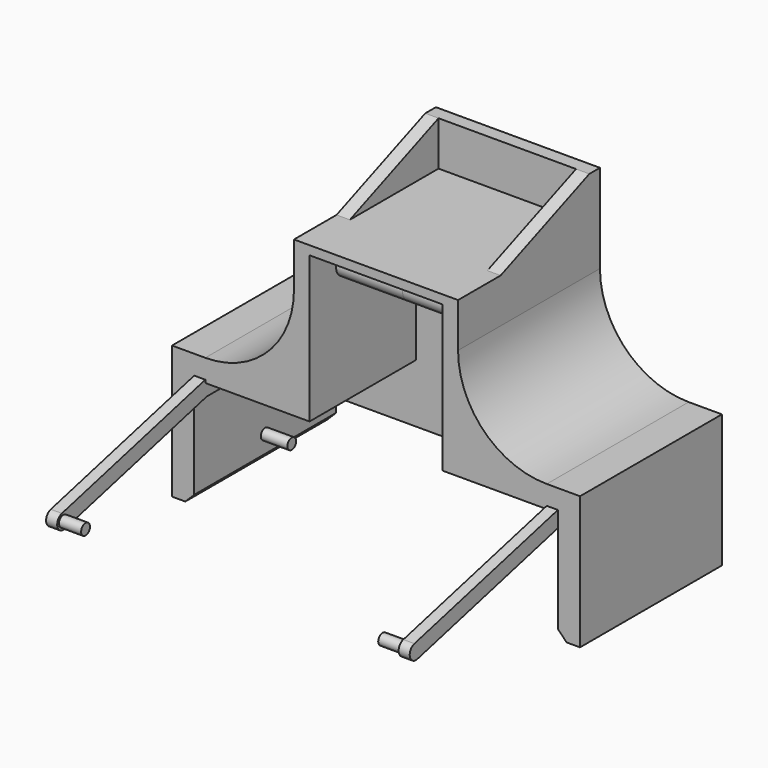
from build123d import *

# Parameters (mm, degrees)
F0_W          = 116.84
F0_H          = 76.2
F1_DEPTH      = 101.6
F3_DEPTH      = 76.2
F5_DEPTH      = 38.1
F5_DEPTH_BACK = 38.1
F6_R          = 3.1115
F7_DEPTH      = 114.3
F7_DEPTH_BACK = 114.3
F9_DEPTH      = 101.601
F11_DEPTH     = 25.401
F12_SIZE      = 5.08
F13_W         = 177.8
F13_H         = 62.1990481529
F14_DEPTH     = 76.2
F15_W         = 93.98
F15_H         = 7.62
F16_DEPTH     = 25.4
F18_DEPTH     = 7.62
F20_DEPTH     = 7.62
F21_R         = 3.175
F22_DEPTH     = 6.35
F23_DEPTH     = 19.05


with BuildPart() as f1:
    # F0 (on Front) → F1 (new body)
    with BuildSketch(Plane.XZ):
        with Locations((58.42, 38.1)):
            Rectangle(F0_W, F0_H)
        with Locations((-58.42, 38.1)):
            Rectangle(F0_W, F0_H)
        with Locations((58.42, -38.1)):
            Rectangle(F0_W, F0_H)
        with Locations((-58.42, -38.1)):
            Rectangle(F0_W, F0_H)
    extrude(amount=-F1_DEPTH)

    # F2 (on face) → F3 (cut)
    with BuildSketch(Plane.XZ):
        Polygon((-38.1, -12.7), (-104.14, -12.7), (-104.14, -69.85), (-104.14, -76.2), (104.14, -76.2), (104.14, -69.85), (104.14, -12.7), (38.1, -12.7), (38.1, 63.5), (-38.1, 63.5), align=None)
    extrude(amount=-F3_DEPTH, mode=Mode.SUBTRACT)

    # F4 (on Right) → F5 (cut, two sides)
    with BuildSketch(Plane.YZ) as f5_sk:
        Polygon((0, 71.12), (0, 63.5), (76.2, 63.5), align=None)
    extrude(amount=-F5_DEPTH, mode=Mode.SUBTRACT)
    extrude(f5_sk.sketch, amount=F5_DEPTH_BACK, mode=Mode.SUBTRACT)

    # F6 (on Right) → F7 (join, two sides)
    with BuildSketch(Plane.YZ) as f7_sk:
        with BuildLine():
            ThreePointArc((25.4005372305, 50.8), (29.8906652911, 52.6598719395), (31.7505372305, 57.15))
            ThreePointArc((31.7505372305, 57.15), (20.91040917, 61.6401280605), (25.4005372305, 50.8))
        make_face()
        with Locations((50.8005372305, -41.021)):
            Circle(F6_R)
        with Locations((50.8005372305, -61.087)):
            Circle(F6_R)
    extrude(amount=F7_DEPTH)
    extrude(f7_sk.sketch, amount=-F7_DEPTH_BACK)

    # F8 (on face) → F9 (cut, through all)
    with BuildSketch(Plane.XZ):
        with BuildLine():
            Line((-46.99, 76.2), (-116.84, 76.2))
            Line((-116.84, 76.2), (-116.84, 0))
            Line((-116.84, 0), (-97.79, 0))
            ThreePointArc((-97.79, 0), (-61.8689755157, 14.8789755157), (-46.99, 50.8))
            Line((-46.99, 50.8), (-46.99, 76.2))
        make_face()
        with BuildLine():
            Line((116.84, 0), (116.84, 76.2))
            Line((116.84, 76.2), (46.99, 76.2))
            Line((46.99, 76.2), (46.99, 50.8))
            ThreePointArc((46.99, 50.8), (61.8689755157, 14.8789755157), (97.79, 0))
            Line((97.79, 0), (116.84, 0))
        make_face()
    extrude(amount=-F9_DEPTH, mode=Mode.SUBTRACT)

    # F10 (on face) → F11 (cut, through all)
    with BuildSketch(Plane.XZ.offset(-76.2)):
        Polygon((104.14, -76.2), (104.14, -48.7679988146), (104.14, -46.2279988146), (-104.14, -46.2279988146), (-104.14, -48.7679988146), (-104.14, -76.2), align=None)
    extrude(amount=-F11_DEPTH, mode=Mode.SUBTRACT)

    # F12
    f12_edges = [f1.edges().sort_by_distance(p)[0] for p in [
        (104.14, 50.8, -76.2),
        (-104.14, 50.8, -76.2),
    ]]
    chamfer(f12_edges, length=F12_SIZE)

    # F13 (on Front) → F14 (cut)
    with BuildSketch(Plane.XZ):
        with Locations((0, -55.8045858206)):
            Rectangle(F13_W, F13_H)
    extrude(amount=-F14_DEPTH, mode=Mode.SUBTRACT)

    # F15 (on face) → F16 (join)
    with BuildSketch(Plane.XY.offset(76.2)):
        with Locations((0, 97.79)):
            Rectangle(F15_W, F15_H)
    extrude(amount=F16_DEPTH)

    # F17 (on face) → F18 (join)
    with BuildSketch(Plane.YZ.offset(46.99)):
        Polygon((93.98, 76.2), (93.98, 101.6), (30.48, 76.2), align=None)
    extrude(amount=-F18_DEPTH)

    # F19 (on face) → F20 (join)
    with BuildSketch(Plane(origin=(-46.99, 0, 0), x_dir=(0, -1, 0), z_dir=(-1, 0, 0))):
        Polygon((-30.48, 76.2), (-93.98, 101.6), (-93.98, 76.2), align=None)
    extrude(amount=-F20_DEPTH)

    # F21 (on face) → F22 (join)
    with BuildSketch(Plane.YZ.offset(-104.14)):
        with BuildLine():
            Line((6.0337829095, -9.5307531462), (-1.0780708533, -11.3087165869))
            Line((-1.0780708533, -11.3087165869), (-102.6780708533, -36.7087165869))
            ThreePointArc((-102.6780708533, -36.7087165869), (-105.9122834131, -42.0990708533), (-100.5219291467, -45.3332834131))
            Line((-100.5219291467, -45.3332834131), (0, -20.2028011265))
            Line((0, -20.2028011265), (1.0780708533, -19.9332834131))
            Line((1.0780708533, -19.9332834131), (14.6432286128, -19.9332834131))
            Line((14.6432286128, -19.9332834131), (14.6432286128, -9.5307531462))
            Line((14.6432286128, -9.5307531462), (6.0337829095, -9.5307531462))
        make_face()
        with Locations((-101.6, -41.021)):
            Circle(F21_R, mode=Mode.SUBTRACT)
        with Locations((-101.6, -41.021)):
            Circle(F21_R)
    extrude(amount=F22_DEPTH)

    # F21 (on face) → F23 (join)
    with BuildSketch(Plane.YZ.offset(-104.14)):
        with Locations((-101.6, -41.021)):
            Circle(F21_R)
    extrude(amount=F23_DEPTH)

    # F24: F1 across plane


with BuildPart() as f1_1:
    add(f1.part)
    add(f1.part.mirror(Plane.YZ))


solid = f1_1.part
